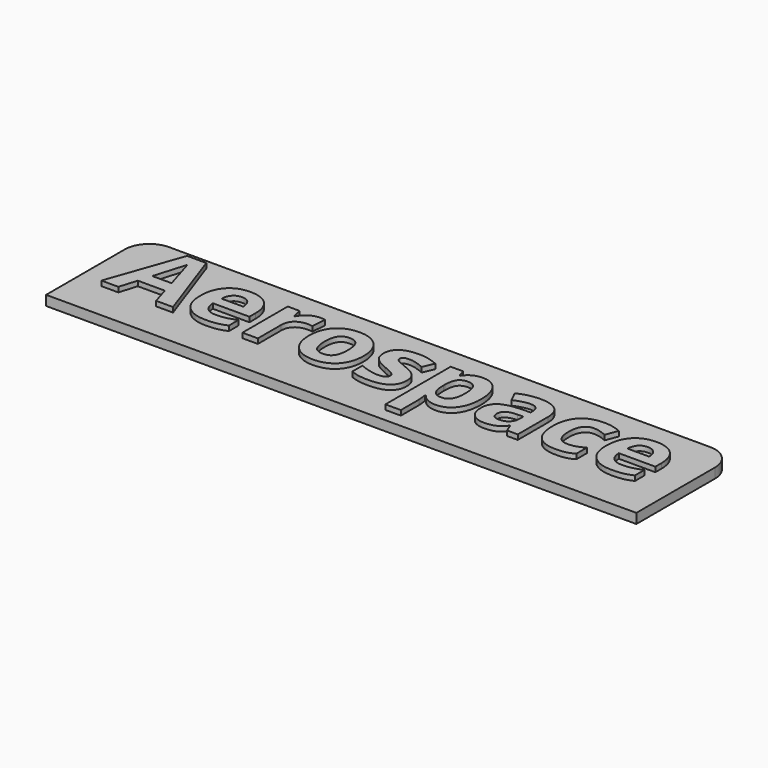
from build123d import *

# Parameters (mm, degrees)
F0_W         = 120
F0_H         = 25
F1_DEPTH     = 2
F2_TEXT_SIZE = 21.0936329588
F3_DEPTH     = 1
F4_R         = 5


# Not quite as in the source:
# - Text() gives the source's letters only with a copy of the font that has no kerning and outlines rounded to 1/6400 em; it was checked with that copy


with BuildPart() as f1:
    # F0 (on Top) → F1 (new body)
    with BuildSketch(Plane.XY):
        Rectangle(F0_W, F0_H)
    extrude(amount=F1_DEPTH)

    # F2 (on face) → F3 (join)
    with BuildSketch(Plane.XY.offset(2)):
        with Locations((-55, -4.6874157303)):
            Text('Aerospace', F2_TEXT_SIZE, font='Open Sans', font_style=FontStyle.BOLD, text_align=(TextAlign.LEFT, TextAlign.BOTTOM))
    extrude(amount=F3_DEPTH)

    # F4
    f4_edges = [f1.edges().sort_by_distance(p)[0] for p in [
        (-60, 12.5, 1),
        (60, 12.5, 1),
    ]]
    fillet(f4_edges, radius=F4_R)


solid = f1.part
